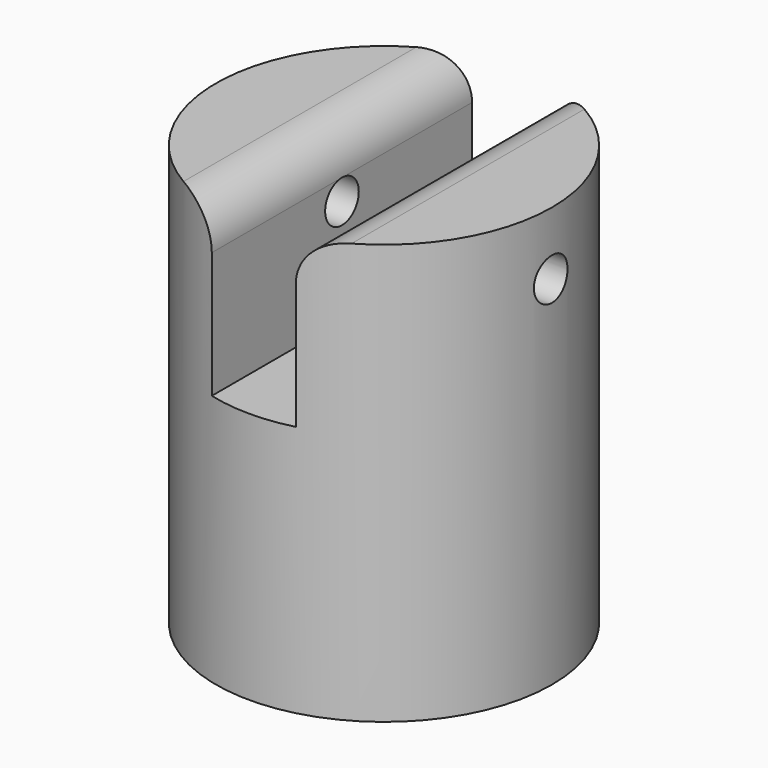
from build123d import *

# Parameters (mm, degrees)
F0_R     = 8
F1_DEPTH = 20
F3_DEPTH = 8
F4_R     = 1
F5_DEPTH = 12.5
F6_R     = 1.99999


# Not quite as in the source:
# - a fillet or chamfer is up to 0.001 mm smaller than in the source, because OpenCascade refuses the exact size


with BuildPart() as f1:
    # F0 (on Top) → F1 (new body)
    with BuildSketch(Plane.XY):
        Circle(F0_R)
    extrude(amount=F1_DEPTH)

    # F2 (on face) → F3 (cut)
    with BuildSketch(Plane.XY.offset(20)):
        with BuildLine():
            ThreePointArc((2, 7.7459666924), (1.0080343399, 7.9362375701), (0, 8))
            ThreePointArc((0, 8), (-1.0080343399, 7.9362375701), (-2, 7.7459666924))
            Line((-2, 7.7459666924), (-2, -7.7459666924))
            ThreePointArc((-2, -7.7459666924), (-1.0080343399, -7.9362375701), (0, -8))
            ThreePointArc((0, -8), (1.0080343399, -7.9362375701), (2, -7.7459666924))
            Line((2, -7.7459666924), (2, 7.7459666924))
        make_face()
    extrude(amount=-F3_DEPTH, mode=Mode.SUBTRACT)

    # F4 (on Right) → F5 (cut, symmetric)
    with BuildSketch(Plane.YZ):
        with Locations((0, 17)):
            Circle(F4_R)
    extrude(amount=F5_DEPTH, both=True, mode=Mode.SUBTRACT)

    # F6 (radius 2 in the source; OpenCascade refuses exactly that, so slightly less here)
    f6_edges = [f1.edges().sort_by_distance(p)[0] for p in [
        (-2, 0, 20),
        (2, 0, 20),
    ]]
    fillet(f6_edges, radius=F6_R)


solid = f1.part
